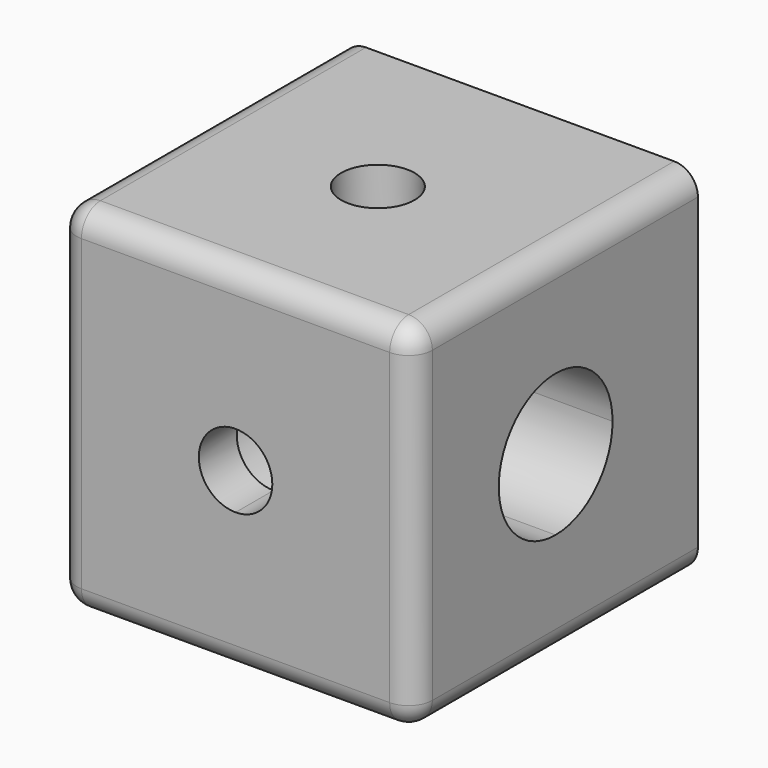
from build123d import *
from build123d import SkipClean  # not in build123d's __all__

# Parameters (mm, degrees)
F0_W      = 15
F0_H      = 15
F1_DEPTH  = 15
F3_DEPTH  = 25
F5_DEPTH  = 25
F7_DEPTH  = 13
F9_DEPTH  = 25
F10_R     = 3
F11_DEPTH = 13
F12_R     = 3
F13_DEPTH = 13
F14_R     = 1


with BuildPart() as f1:
    # F0 (on Top) → F1 (new body)
    with BuildSketch(Plane.XY):
        with Locations((-7.5, 7.5)):
            Rectangle(F0_W, F0_H)
    extrude(amount=F1_DEPTH)

    # F2 (on face) → F3 (cut)
    with BuildSketch(Plane.XZ):
        with BuildLine():
            ThreePointArc((-7.5, 5.95), (-6.4039844892, 6.4039844892), (-5.95, 7.5))
            ThreePointArc((-5.95, 7.5), (-8.5960155108, 8.5960155108), (-7.5, 5.95))
        make_face()
    extrude(amount=-F3_DEPTH, mode=Mode.SUBTRACT)

    # F4 (on face) → F5 (cut)
    with BuildSketch(Plane.XY.offset(15)):
        with BuildLine():
            ThreePointArc((-7.5, 5.95), (-6.4039844892, 6.4039844892), (-5.95, 7.5))
            ThreePointArc((-5.95, 7.5), (-8.5960155108, 8.5960155108), (-7.5, 5.95))
        make_face()
    extrude(amount=-F5_DEPTH, mode=Mode.SUBTRACT)

    # F6 (on face) → F7 (cut)
    with BuildSketch(Plane.YZ):
        with BuildLine():
            ThreePointArc((7.5, 4.5), (9.6213203436, 5.3786796564), (10.5, 7.5))
            ThreePointArc((10.5, 7.5), (5.3786796564, 9.6213203436), (7.5, 4.5))
        make_face()
    with SkipClean():  # cleaning this boolean's faces spoils the solid; the shape is the same uncleaned
        extrude(amount=-F7_DEPTH, mode=Mode.SUBTRACT)

    # F8 (on face) → F9 (cut)
    with BuildSketch(Plane(origin=(-15, 0, 0), x_dir=(0, -1, 0), z_dir=(-1, 0, 0))):
        with BuildLine():
            ThreePointArc((-7.5, 5.95), (-6.4039844892, 6.4039844892), (-5.95, 7.5))
            ThreePointArc((-5.95, 7.5), (-8.5960155108, 8.5960155108), (-7.5, 5.95))
        make_face()
    with SkipClean():  # cleaning this boolean's faces spoils the solid; the shape is the same uncleaned
        extrude(amount=-F9_DEPTH, mode=Mode.SUBTRACT)

    # F10 (on face) → F11 (cut)
    with BuildSketch(Plane(origin=(0, 15, 0), x_dir=(-1, 0, 0), z_dir=(0, 1, 0))):
        with Locations((7.5, 7.5)):
            Circle(F10_R)
    extrude(amount=-F11_DEPTH, mode=Mode.SUBTRACT)

    # F12 (on face) → F13 (cut)
    with BuildSketch(Plane(origin=(0, 0, 0), x_dir=(1, 0, 0), z_dir=(0, 0, -1))):
        with Locations((-7.5, -7.5)):
            Circle(F12_R)
    extrude(amount=-F13_DEPTH, mode=Mode.SUBTRACT)

    # F14
    f14_edges = [f1.edges().sort_by_distance(p)[0] for p in [
        (-15, 0, 7.5),
        (-7.5, 0, 0),
        (0, 0, 7.5),
        (-7.5, 0, 15),
        (-15, 7.5, 0),
        (-15, 7.5, 15),
        (0, 7.5, 15),
        (0, 7.5, 0),
    ]]
    fillet(f14_edges, radius=F14_R)


solid = f1.part
